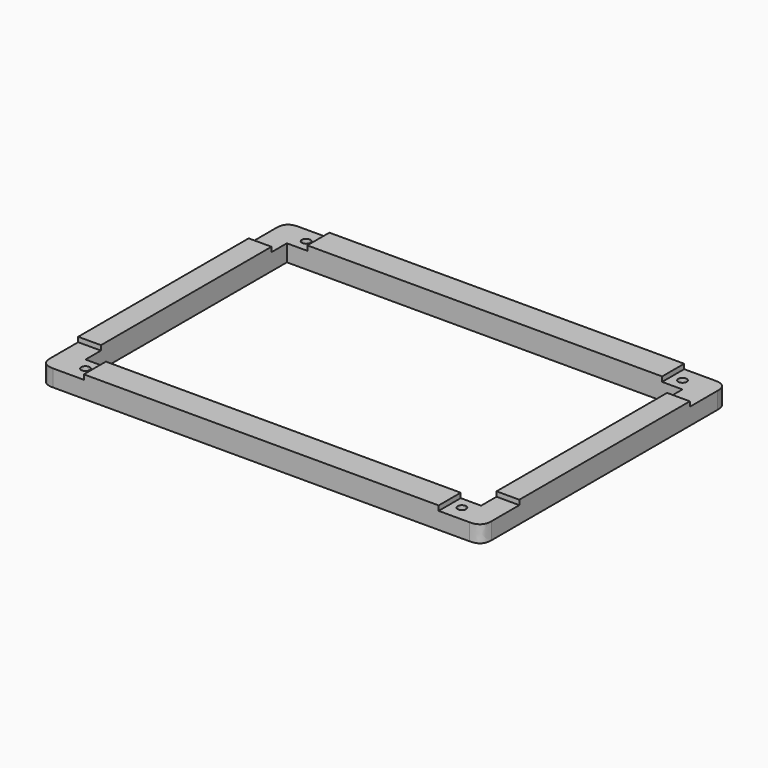
from build123d import *

# Parameters (mm, degrees)
F0_W        = 184
F0_H        = 128
F1_DEPTH    = 7
F2_W        = 165
F2_H        = 105
F3_DEPTH    = 7
F4_W        = 74
F4_H        = 11.5
F5_DEPTH    = 2
F6_T1_DEPTH = 32.4
F7_W        = 9.5
F7_H        = 44.45
F8_DEPTH    = 2
F10_DEPTH   = 7
F12_DEPTH   = 7


# Not quite as in the source:
# - a fillet or chamfer that OpenCascade refuses, or shapes differently, is made with other operations: its cross-section is extruded or revolved along the edge and cut away or added
# - a pattern or mirror of a feature is missing from the dataset's text; its kind, count and spacing are read off the source's solid


with BuildPart() as f1:
    # F0 (on Top) → F1 (new body)
    with BuildSketch(Plane.XY):
        Rectangle(F0_W, F0_H)
    extrude(amount=F1_DEPTH)

    # F2 (on face) → F3 (cut, through all)
    with BuildSketch(Plane.XY.offset(7)):
        Rectangle(F2_W, F2_H)
    extrude(amount=-F3_DEPTH, mode=Mode.SUBTRACT)

    # F4 (on face) → F5 (join)
    with BuildSketch(Plane.XY.offset(7)):
        with Locations((-37, 58.25)):
            Rectangle(F4_W, F4_H)
        with Locations((37, 58.25)):
            Rectangle(F4_W, F4_H)
        with Locations((-37, -58.25)):
            Rectangle(F4_W, F4_H)
        with Locations((37, -58.25)):
            Rectangle(F4_W, F4_H)
    extrude(amount=F5_DEPTH)

    # F6: fillet of radius 5.08 on 4 edges, made by hand

    # F6_s2 → F6_t1 (cut)
    with BuildSketch(Plane.XY.offset(-12.7)):
        with BuildLine():
            add(Edge.make_bspline(
                [(92, -58.92), (92, -64), (86.92, -64)],
                knots=[0, 0, 0, 1, 1, 1], degree=2, weights=[1, 1, 1]))
            Line((86.92, -64), (92, -64))
            Line((92, -64), (92, -58.92))
        make_face()
        with BuildLine():
            add(Edge.make_bspline(
                [(92, 58.92), (92, 64), (86.92, 64)],
                knots=[0, 0, 0, 1, 1, 1], degree=2, weights=[1, 1, 1]))
            Line((86.92, 64), (92, 64))
            Line((92, 64), (92, 58.92))
        make_face()
        with BuildLine():
            add(Edge.make_bspline(
                [(-86.92, 64), (-92, 64), (-92, 58.92)],
                knots=[0, 0, 0, 1, 1, 1], degree=2, weights=[1, 1, 1]))
            Line((-92, 58.92), (-92, 64))
            Line((-92, 64), (-86.92, 64))
        make_face()
        with BuildLine():
            add(Edge.make_bspline(
                [(-86.92, -64), (-92, -64), (-92, -58.92)],
                knots=[0, 0, 0, 1, 1, 1], degree=2, weights=[1, 1, 1]))
            Line((-92, -58.92), (-92, -64))
            Line((-92, -64), (-86.92, -64))
        make_face()
    extrude(amount=F6_T1_DEPTH, mode=Mode.SUBTRACT)

    # F7 (on face) → F8 (join)
    with BuildSketch(Plane.XY.offset(7)):
        with Locations((87.25, -22.225)):
            Rectangle(F7_W, F7_H)
        with Locations((87.25, 22.225)):
            Rectangle(F7_W, F7_H)
    f8 = extrude(amount=F8_DEPTH)

    # F8_copies: F8 across plane
    add(f8.mirror(Plane(origin=(0, 0, 0), x_dir=(0, 0, -1), z_dir=(-1, 0, 0))))

    # F9 (on face) → F10 (cut, through all)
    with BuildSketch(Plane.XY.offset(7)):
        with BuildLine():
            ThreePointArc((80.25, 57.5), (77.2625631329, 58.7374368671), (78.5, 55.75))
            ThreePointArc((78.5, 55.75), (79.7374368671, 56.2625631329), (80.25, 57.5))
        make_face()
    f10 = extrude(amount=-F10_DEPTH, mode=Mode.SUBTRACT)

    # F10_copies: F10 across plane
    add(f10.mirror(Plane(origin=(0, 0, 0), x_dir=(0, 0, -1), z_dir=(-1, 0, 0))), mode=Mode.SUBTRACT)

    # F11 (on face) → F12 (cut, through all)
    with BuildSketch(Plane(origin=(0, 0, 0), x_dir=(1, 0, 0), z_dir=(0, 0, -1))):
        with BuildLine():
            ThreePointArc((-76.75, 57.5), (-79.7374368671, 58.7374368671), (-78.5, 55.75))
            ThreePointArc((-78.5, 55.75), (-77.2625631329, 56.2625631329), (-76.75, 57.5))
        make_face()
        with BuildLine():
            ThreePointArc((80.25, 57.5), (77.2625631329, 58.7374368671), (78.5, 55.75))
            ThreePointArc((78.5, 55.75), (79.7374368671, 56.2625631329), (80.25, 57.5))
        make_face()
    extrude(amount=-F12_DEPTH, mode=Mode.SUBTRACT)


solid = f1.part
